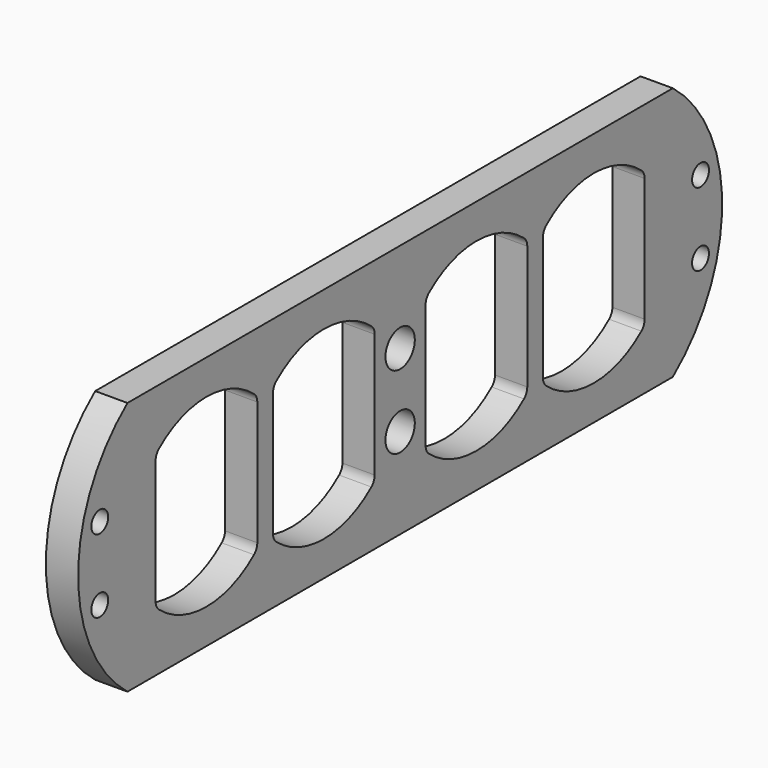
from build123d import *

# Parameters (mm, degrees)
F0_R     = 1.8288
F0_R_2   = 3.175
F1_DEPTH = 5.588
F2_R     = 2


# Not quite as in the source:
# - a feature names something its author has since deleted; it is built from what else it names


with BuildPart() as f1:
    # F0 (on Right) → F1 (new body)
    with BuildSketch(Plane.YZ):
        with BuildLine():
            ThreePointArc((59, -22), (69.6794919243, 0), (59, 22))
            Line((59, 22), (-59, 22))
            ThreePointArc((-59, 22), (-69.6794919243, 0), (-59, -22))
            Line((-59, -22), (59, -22))
        make_face()
        with Locations((-65, -6.35)):
            Circle(F0_R, mode=Mode.SUBTRACT)
        with Locations((0, -6.35)):
            Circle(F0_R_2, mode=Mode.SUBTRACT)
        with Locations((65, -6.35)):
            Circle(F0_R, mode=Mode.SUBTRACT)
        with BuildLine():
            ThreePointArc((-30.91, -11.6189500386), (-41.91, -16), (-52.91, -11.6189500386))
            Line((-52.91, -11.6189500386), (-52.91, 11.6189500386))
            ThreePointArc((-52.91, 11.6189500386), (-41.91, 16), (-30.91, 11.6189500386))
            Line((-30.91, 11.6189500386), (-30.91, -11.6189500386))
        make_face(mode=Mode.SUBTRACT)
        with Locations((-65, 6.35)):
            Circle(F0_R, mode=Mode.SUBTRACT)
        with BuildLine():
            ThreePointArc((-27.51, 11.6189500386), (-16.51, 16), (-5.51, 11.6189500386))
            Line((-5.51, 11.6189500386), (-5.51, -11.6189500386))
            ThreePointArc((-5.51, -11.6189500386), (-16.51, -16), (-27.51, -11.6189500386))
            Line((-27.51, -11.6189500386), (-27.51, 11.6189500386))
        make_face(mode=Mode.SUBTRACT)
        with BuildLine():
            ThreePointArc((27.51, -11.6189500386), (16.51, -16), (5.51, -11.6189500386))
            Line((5.51, -11.6189500386), (5.51, 11.6189500386))
            ThreePointArc((5.51, 11.6189500386), (16.51, 16), (27.51, 11.6189500386))
            Line((27.51, 11.6189500386), (27.51, -11.6189500386))
        make_face(mode=Mode.SUBTRACT)
        with Locations((0, 6.35)):
            Circle(F0_R_2, mode=Mode.SUBTRACT)
        with BuildLine():
            ThreePointArc((52.91, -11.6189500386), (41.91, -16), (30.91, -11.6189500386))
            Line((30.91, -11.6189500386), (30.91, 11.6189500386))
            ThreePointArc((30.91, 11.6189500386), (41.91, 16), (52.91, 11.6189500386))
            Line((52.91, 11.6189500386), (52.91, -11.6189500386))
        make_face(mode=Mode.SUBTRACT)
        with Locations((65, 6.35)):
            Circle(F0_R, mode=Mode.SUBTRACT)
    extrude(amount=F1_DEPTH)

    # F2
    f2_edges = [f1.edges().sort_by_distance(p)[0] for p in [
        (2.794, -5.51, 11.61895),
        (2.794, 52.91, 11.61895),
        (2.794, 5.51, -11.61895),
        (2.794, 5.51, 11.61895),
        (2.794, -52.91, -11.61895),
        (2.794, -52.91, 11.61895),
        (2.794, -5.51, -11.61895),
        (2.794, 52.91, -11.61895),
        (2.794, -30.91, -11.61895),
        (2.794, -30.91, 11.61895),
        (2.794, -27.51, -11.61895),
        (2.794, -27.51, 11.61895),
        (2.794, 27.51, 11.61895),
        (2.794, 27.51, -11.61895),
        (2.794, 30.91, 11.61895),
        (2.794, 30.91, -11.61895),
    ]]
    fillet(f2_edges, radius=F2_R)


solid = f1.part
